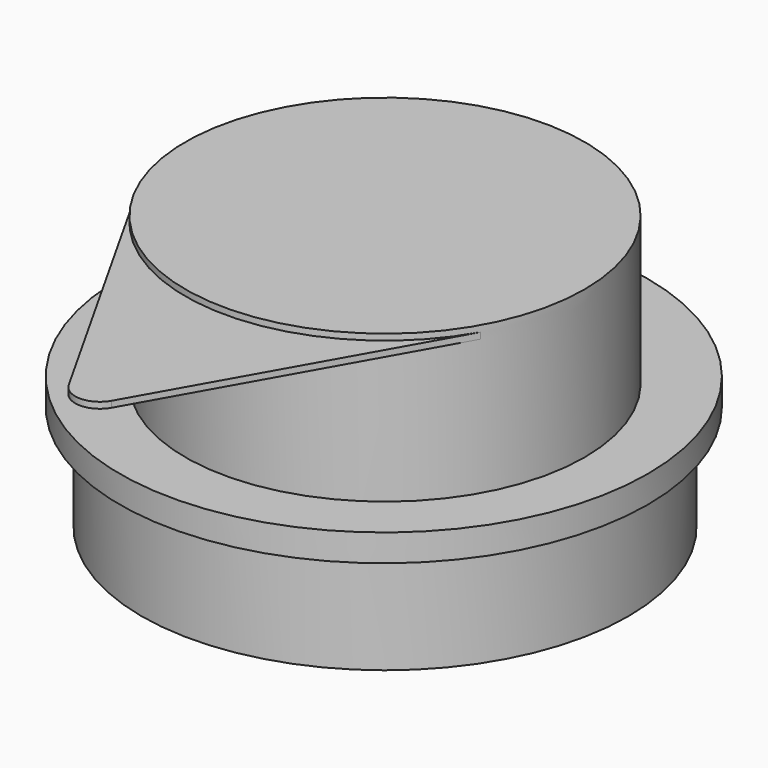
from build123d import *

# Parameters (mm, degrees)
F0_R      = 19.75
F1_DEPTH  = 8
F2_R      = 21.425
F3_DEPTH  = 2.2
F4_R      = 16.2
F5_DEPTH  = 12
F10_DEPTH = 0.5


# Not quite as in the source:
# - the program builds the solid bodies; features that only make, move or delete a surface that nothing else refers to are left out


with BuildPart() as f1:
    # F0 (on Top) → F1 (new body)
    with BuildSketch(Plane.XY):
        Circle(F0_R)
    extrude(amount=F1_DEPTH)

    # F2 (on face) → F3 (join)
    with BuildSketch(Plane.XY.offset(8)):
        with Locations((-0.6810527993, 0.7295852411)):
            Circle(F2_R)
    extrude(amount=F3_DEPTH)

    # F4 (on face) → F5 (join)
    with BuildSketch(Plane.XY.offset(10.2)):
        Circle(F4_R)
    extrude(amount=F5_DEPTH)

    # F7 (on offset) → F10 (join)
    with BuildSketch(Plane.XY.offset(21.2)):
        with BuildLine():
            ThreePointArc((14.1136150197, -7.9527272727), (15.6697250027, -4.1109267009), (16.2, 0))
            ThreePointArc((16.2, 0), (-4.1109267009, 15.6697250027), (-14.1136150197, -7.9527272727))
            ThreePointArc((-14.1136150197, -7.9527272727), (0, -16.2), (14.1136150197, -7.9527272727))
        make_face()
        with BuildLine():
            ThreePointArc((14.1136150197, -7.9527272727), (0, -16.2), (-14.1136150197, -7.9527272727))
            Line((-14.1136150197, -7.9527272727), (-1.7424216074, -29.9077441077))
            ThreePointArc((-1.7424216074, -29.9077441077), (0, -30.9259259259), (1.7424216074, -29.9077441077))
            Line((1.7424216074, -29.9077441077), (14.1136150197, -7.9527272727))
        make_face()
    extrude(amount=F10_DEPTH)


solid = f1.part
